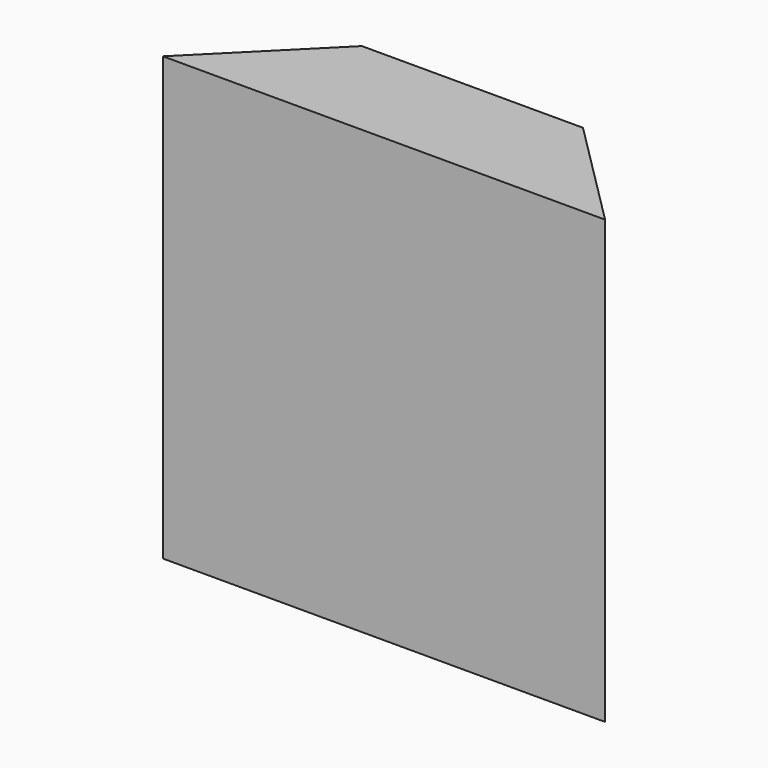
from build123d import *

# Parameters (mm, degrees)
F0_W     = 100
F0_H     = 100
F1_DEPTH = 25
F2_SIZE  = 24.99999


# Not quite as in the source:
# - a fillet or chamfer is up to 0.001 mm smaller than in the source, because OpenCascade refuses the exact size


with BuildPart() as f1:
    # F0 (on Front) → F1 (new body)
    with BuildSketch(Plane.XZ):
        Rectangle(F0_W, F0_H)
    extrude(amount=-F1_DEPTH)

    # F2 (size 25 in the source; OpenCascade refuses exactly that, so slightly less here)
    f2_edges = [f1.edges().sort_by_distance(p)[0] for p in [
        (50, 25, 0),
        (-50, 25, 0),
    ]]
    chamfer(f2_edges, length=F2_SIZE)


solid = f1.part
